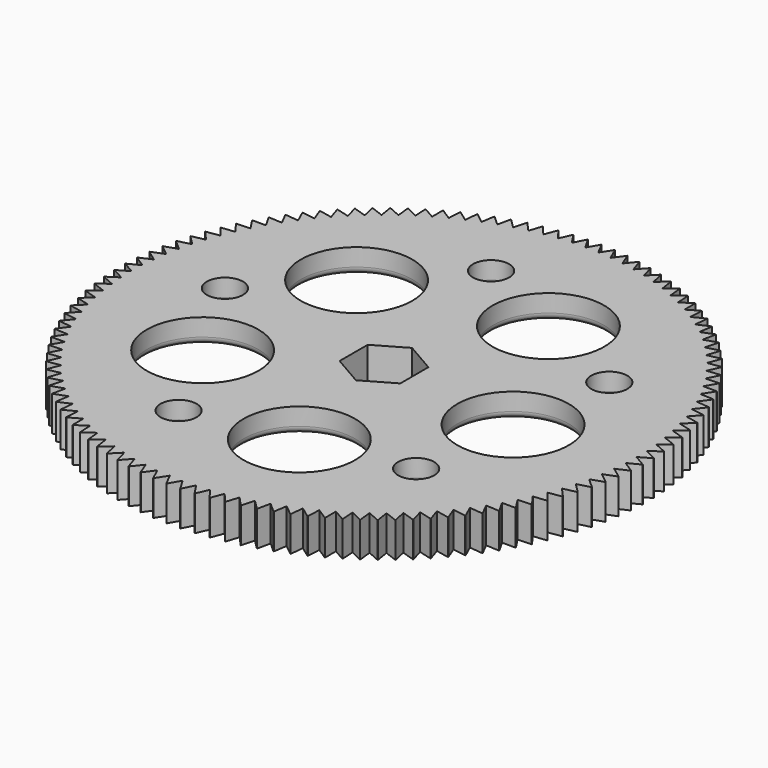
from build123d import *

# Parameters (mm, degrees)
F0_R             = 37.647
F0_R_2           = 7.115222554
F1_DEPTH         = 5
F4_DEPTH         = 5
F4_COPIES_COUNT  = 120
F6_R             = 35
F6_R_2           = 7.115222554
F8_DEPTH         = 1.5
F10_R            = 7.963
F10_R_2          = 2.5785
F11_DEPTH        = 10
F11_COPIES_COUNT = 5
F12_R            = 1


# Not quite as in the source:
# - a fillet or chamfer that OpenCascade refuses, or shapes differently, is made with other operations: its cross-section is extruded or revolved along the edge and cut away or added
# - a pattern or mirror of a feature is missing from the dataset's text; its kind, count and spacing are read off the source's solid


with BuildPart() as f1:
    # F0 (on Top) → F1 (new body)
    with BuildSketch(Plane.XY):
        Circle(F0_R)
        Circle(F0_R_2, mode=Mode.SUBTRACT)
        Circle(F0_R_2)
        Polygon((4.3301270189, -2.5), (0, -5), (-4.3301270189, -2.5), (-4.3301270189, 2.5), (0, 5), (4.3301270189, 2.5), align=None, mode=Mode.SUBTRACT)
    extrude(amount=F1_DEPTH)

    # F3 (on Top) → F4 (cut)
    with BuildSketch(Plane.XY):
        Polygon((21.4533342869, -31.5427972281), (23.4733408366, -30.0698499991), (21.187727843, -29.0569466258), align=None)
    f4 = extrude(amount=F4_DEPTH, mode=Mode.SUBTRACT)

    # F4_copies: F4 ×120 about axis
    f4_copies_axis = Axis((0, 0, 0), (0, 0, 1))
    for i in range(1, F4_COPIES_COUNT):
        add(f4.rotate(f4_copies_axis, i * 360 / F4_COPIES_COUNT), mode=Mode.SUBTRACT)

    # F6 (on face) → F8 (cut)
    with BuildSketch(Plane.XY):
        Circle(F6_R)
        Circle(F6_R_2, mode=Mode.SUBTRACT)
    extrude(amount=F8_DEPTH, mode=Mode.SUBTRACT)

    # F9: fillet of radius 5 on 2 edges, made by hand

    # F9_s1 → F9_t2 (revolve)
    with BuildSketch(Plane.XZ):
        with BuildLine():
            ThreePointArc((35, 0), (33.3657774588, 1.1097722286), (31.4292857857, 1.5))
            Line((31.4292857857, 1.5), (35, 1.5))
            Line((35, 1.5), (35, 0))
        make_face()
    revolve(axis=Axis((0, 0, 1.5), (0, 0, 1)))

    # F9_s3 → F9_t4 (revolve)
    with BuildSketch(Plane.XZ):
        with BuildLine():
            ThreePointArc((10.6859367683, 1.5), (8.7494450952, 1.1097722286), (7.115222554, 0))
            Line((7.115222554, 0), (7.115222554, 1.5))
            Line((7.115222554, 1.5), (10.6859367683, 1.5))
        make_face()
    revolve(axis=Axis((0, 0, 1.5), (0, 0, 1)))

    # F10 (on face) → F11 (cut)
    with BuildSketch(Plane.XY):
        with Locations((-17.8716722876, -10.005151853)):
            Circle(F10_R)
        with Locations((-10.8700487763, -23.0378154665)):
            Circle(F10_R_2)
    f11 = extrude(amount=F11_DEPTH, mode=Mode.SUBTRACT)

    # F11_copies: F11 ×5 about axis
    f11_copies_axis = Axis((0, 0, 0), (0, 0, 1))
    for i in range(1, F11_COPIES_COUNT):
        add(f11.rotate(f11_copies_axis, i * 360 / F11_COPIES_COUNT), mode=Mode.SUBTRACT)

    # F12
    f12_edges = [f1.edges().sort_by_distance(p)[0] for p in [
        (-25.834672, -10.005152, 1.5),
        (-13.448549, -23.037815, 1.5),
        (1.532112, -27.661995, 1.5),
        (17.754434, -19.909406, 1.5),
        (26.78157, -7.090901, 1.5),
        (-26.066095, 5.671253, 1.5),
        (-17.498818, 21.478471, 1.5),
        (-2.661184, 26.542843, 1.5),
        (24.421393, 10.733126, 1.5),
        (15.019808, 23.279577, 1.5),
    ]]
    fillet(f12_edges, radius=F12_R)


solid = f1.part
